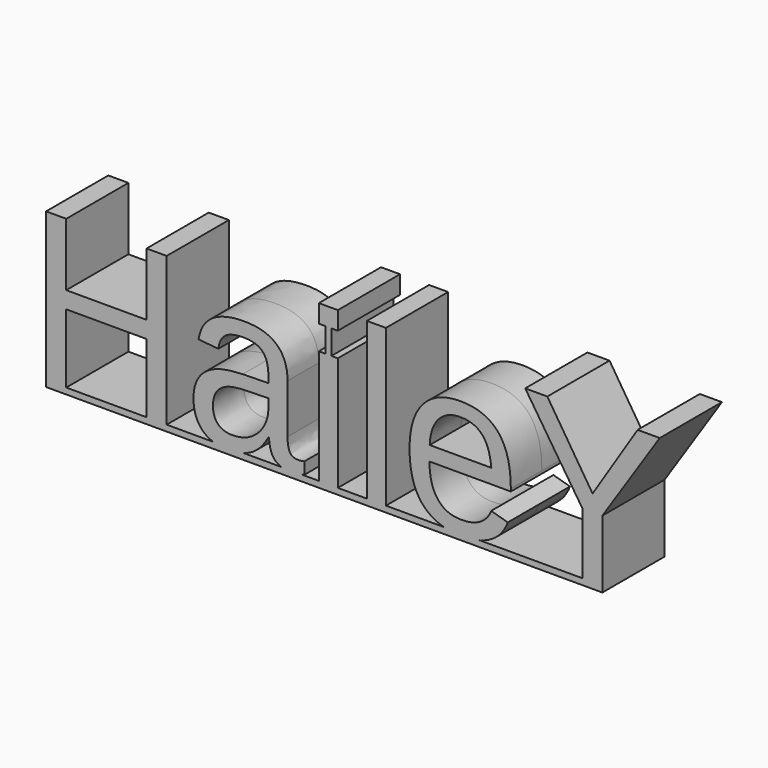
from build123d import *

# Parameters (mm, degrees)
F0_TEXT_SIZE = 35.2777777778
F1_DEPTH     = 6.35
F2_W         = 90.8788628472
F2_H         = 12.7
F3_DEPTH     = 1
F4_W         = 1
F4_H         = 3.9632378472
F5_DEPTH     = 12.7


# Not quite as in the source:
# - Text() gives the source's letters only with a copy of the font that has no kerning and outlines rounded to 1/6400 em; it was checked with that copy


with BuildPart() as f1:
    # F0 (on Front) → F1 (new body, symmetric)
    with BuildSketch(Plane.XZ):
        with Locations((-52.7953993056, 0)):
            Text('HaileY', F0_TEXT_SIZE, font='Arimo', text_align=(TextAlign.LEFT, TextAlign.BOTTOM))
    extrude(amount=F1_DEPTH, both=True)

    # F2 (on Top) → F3 (join)
    with BuildSketch(Plane.XY):
        with Locations((-4.4620876736, 0)):
            Rectangle(F2_W, F2_H)
    extrude(amount=-F3_DEPTH)

    # F4 (on face) → F5 (join, through all)
    with BuildSketch(Plane.XZ.offset(6.35)):
        Polygon((-5.3412760417, 22.5998263889), (-4.2896050347, 22.5998263889), (-3.2896050347, 22.5998263889), (-2.2379340278, 22.5998263889), (-2.2379340278, 25.5653645833), (-5.3412760417, 25.5653645833), align=None)
        with Locations((-3.7896050347, 20.6182074653)):
            Rectangle(F4_W, F4_H)
    extrude(amount=-F5_DEPTH)


solid = f1.part
